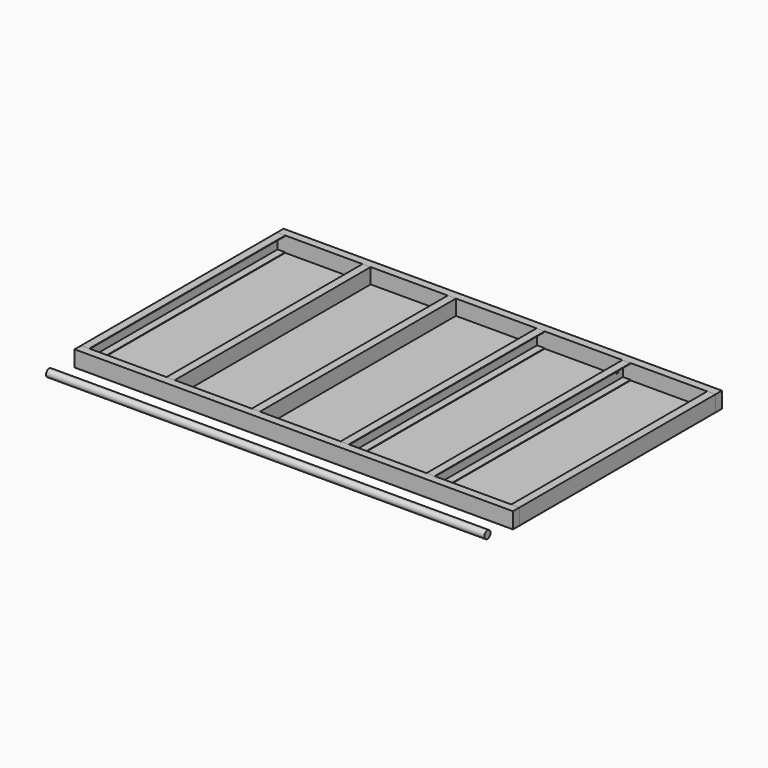
from build123d import *

# Parameters (mm, degrees)
F1_DEPTH  = 512.5
F3_W      = 1720
F3_H      = 1025
F4_DEPTH  = 3
F12_R     = 5
F13_DEPTH = 1000
F15_R     = 15
F16_DEPTH = 1720
F17_W     = 32
F17_H     = 60
F18_DEPTH = 1720


with BuildPart() as f1:
    # F0 (on Front) → F1 (new body, symmetric)
    with BuildSketch(Plane.XZ):
        Polygon((0, 60), (0, 0), (32, 0), (32, 2), (2, 2), (2, 58), (32, 58), (32, 60), align=None)
    extrude(amount=F1_DEPTH, both=True)


with BuildPart() as f1_1:
    # F2: moved
    add(f1.part.moved(Location((158.25, 0, 0))))


with BuildPart() as f4:
    # F3 (on Top) → F4 (new body)
    with BuildSketch(Plane.XY):
        Rectangle(F3_W, F3_H)
    extrude(amount=-F4_DEPTH)


with BuildPart() as f5_1:
    # F5: copy of F1
    add(f1_1.part.moved(Location((337, 0, 0))))


with BuildPart() as f10_1:
    # F10: instance of F5_1
    add(f5_1.part.mirror(Plane.YZ.offset(677.625)))


with BuildPart() as f11_1:
    # F11: instance of F1
    add(f1_1.part.mirror(Plane.YZ))


with BuildPart() as f11_2:
    # F11: instance of F10_1
    add(f10_1.part.mirror(Plane.YZ))


with BuildPart() as f5_1_1:
    add(f5_1.part)

    # F12 (on face) → F13 (cut, symmetric)
    with BuildSketch(Plane(origin=(495.25, 0, 0), x_dir=(0, -1, 0), z_dir=(-1, 0, 0))):
        with Locations((-452.5, 30)):
            Circle(F12_R)
    extrude(amount=F13_DEPTH, both=True, mode=Mode.SUBTRACT)


with BuildPart() as f14_1:
    # F14: copy of F11_1
    add(f11_1.part.moved(Location((-334.5, 0, 0))))


with BuildPart() as f16:
    # F15 (on face) → F16 (new body, through all)
    with BuildSketch(Plane.YZ.offset(860)):
        with Locations((-637.5, 30)):
            Circle(F15_R)
    extrude(amount=-F16_DEPTH)


with BuildPart() as f18:
    # F17 (on face) → F18 (new body, through all)
    with BuildSketch(Plane.YZ.offset(860)):
        with Locations((496.5, 30)):
            Rectangle(F17_W, F17_H)
    extrude(amount=-F18_DEPTH)


with BuildPart() as f19_1:
    # F19: instance of F18
    add(f18.part.mirror(Plane.XZ))


solid = Compound([f1_1.part, f4.part, f10_1.part, f11_1.part, f11_2.part, f5_1_1.part, f14_1.part, f16.part, f18.part, f19_1.part])
